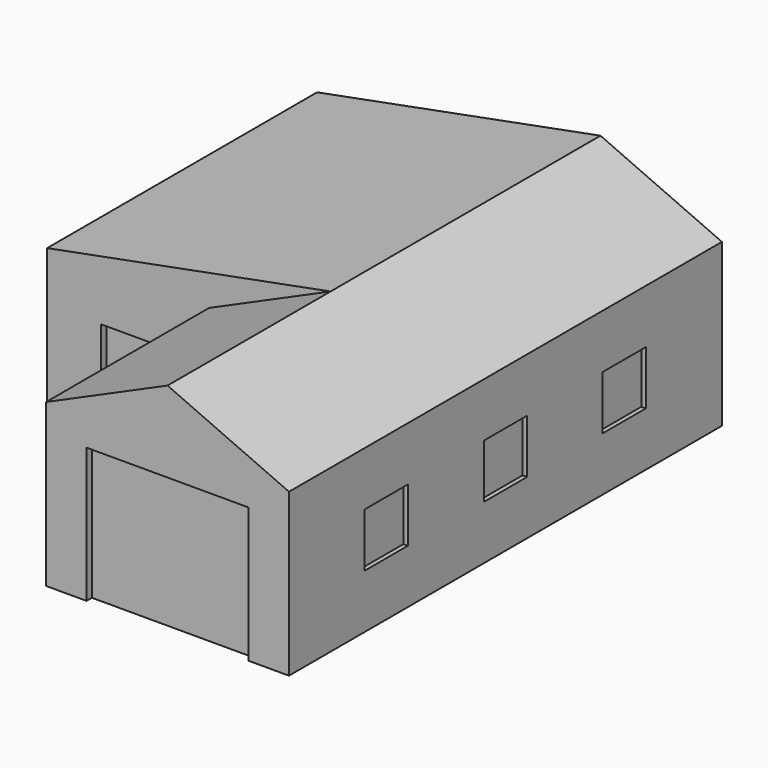
from build123d import *

# Parameters (mm, degrees)
F1_DEPTH      = 12192
F2_W          = 7620
F2_H          = 3657.6
F3_DEPTH      = 3657.6
F3_DEPTH_BACK = 2743.2
F4_DEPTH      = 30.48
F5_W          = 3657.6
F5_H          = 3048
F6_DEPTH      = 152.4
F7_W          = 3048
F7_H          = 3048
F8_DEPTH      = 152.4
F9_W          = 1219.2
F9_H          = 2438.4
F10_DEPTH     = 152.4
F11_W         = 1219.2
F11_H         = 1219.2
F12_DEPTH     = 100.584
F13_W         = 1219.2
F13_H         = 1219.2
F14_DEPTH     = 100.584
F15_W         = 1219.2
F15_H         = 1219.2
F16_DEPTH     = 100.584
F18_DEPTH     = 7620


with BuildPart() as f1:
    # F0 (on Front) → F1 (new body)
    with BuildSketch(Plane.XZ):
        Polygon((0, 3657.6), (0, 0), (5486.4, 0), (5486.4, 3657.6), (2743.2, 4876.8), align=None)
    extrude(amount=F1_DEPTH)

    # F2 (on face) → F3 (join, two sides)
    with BuildSketch(Plane(origin=(0, 0, 0), x_dir=(0, -1, 0), z_dir=(-1, 0, 0))) as f3_sk:
        with Locations((3810, 1828.8)):
            Rectangle(F2_W, F2_H)
    extrude(amount=F3_DEPTH)
    extrude(f3_sk.sketch, amount=-F3_DEPTH_BACK)

    # F4 (add): a face of the model
    f4_faces = [f1.faces().sort_by_distance(p)[0] for p in [
        (2743.2, -12192, 2148.1142857143),
    ]]
    extrude(f4_faces, amount=F4_DEPTH)

    # F5 (on face) → F6 (cut)
    with BuildSketch(Plane.XZ.offset(12222.48)):
        with Locations((2743.2, 1524)):
            Rectangle(F5_W, F5_H)
    extrude(amount=-F6_DEPTH, mode=Mode.SUBTRACT)

    # F7 (on face) → F8 (cut)
    with BuildSketch(Plane(origin=(-3657.6, 0, 0), x_dir=(0, -1, 0), z_dir=(-1, 0, 0))):
        with Locations((3810, 1524)):
            Rectangle(F7_W, F7_H)
    extrude(amount=-F8_DEPTH, mode=Mode.SUBTRACT)

    # F9 (on face) → F10 (cut)
    with BuildSketch(Plane.XZ.offset(7620)):
        with Locations((-1828.8, 1319.784)):
            Rectangle(F9_W, F9_H)
    extrude(amount=-F10_DEPTH, mode=Mode.SUBTRACT)

    # F11 (on face) → F12 (cut)
    with BuildSketch(Plane.YZ.offset(5486.4)):
        with Locations((-9479.28, 1828.8)):
            Rectangle(F11_W, F11_H)
        with Locations((-6111.24, 1828.8)):
            Rectangle(F11_W, F11_H)
        with Locations((-2758.44, 1828.8)):
            Rectangle(F11_W, F11_H)
    extrude(amount=-F12_DEPTH, mode=Mode.SUBTRACT)

    # F13 (on face) → F14 (cut)
    with BuildSketch(Plane(origin=(0, 0, 0), x_dir=(-1, 0, 0), z_dir=(0, 1, 0))):
        with Locations((-2743.2, 1828.8)):
            Rectangle(F13_W, F13_H)
        with Locations((1524, 1828.8)):
            Rectangle(F13_W, F13_H)
    extrude(amount=-F14_DEPTH, mode=Mode.SUBTRACT)

    # F15 (on face) → F16 (cut)
    with BuildSketch(Plane(origin=(0, 0, 0), x_dir=(0, -1, 0), z_dir=(-1, 0, 0))):
        with Locations((9936.48, 1828.8)):
            Rectangle(F15_W, F15_H)
    extrude(amount=-F16_DEPTH, mode=Mode.SUBTRACT)

    # F17 (on face) → F18 (join)
    with BuildSketch(Plane(origin=(0, 0, 0), x_dir=(-1, 0, 0), z_dir=(0, 1, 0))):
        Polygon((3657.6, 3657.6), (-2743.2, 4876.8), (0, 3657.6), align=None)
    extrude(amount=-F18_DEPTH)


solid = f1.part
